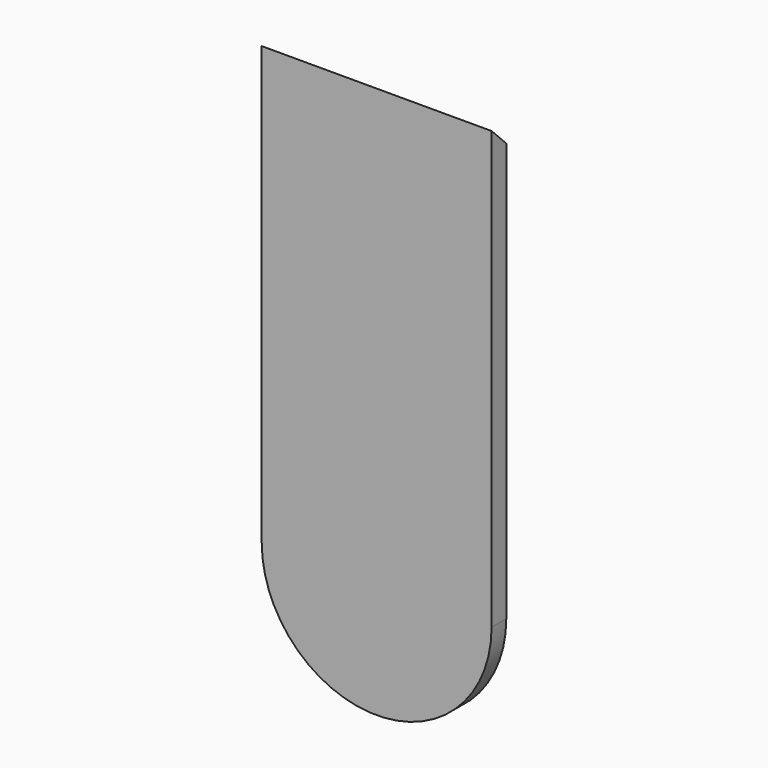
from build123d import *

# Parameters (mm, degrees)
F1_DEPTH = 20
F0_W     = 250
F0_H     = 475
F2_DEPTH = 20
F3_SIZE  = 19.99999


# Not quite as in the source:
# - a fillet or chamfer is up to 0.001 mm smaller than in the source, because OpenCascade refuses the exact size


with BuildPart() as f1:
    # F0 (on Front) → F1 (new body)
    with BuildSketch(Plane.XZ):
        with BuildLine():
            Line((123.788267374, 0), (-126.211732626, 0))
            ThreePointArc((-126.211732626, 0), (-1.211732626, -125), (123.788267374, 0))
        make_face()
    extrude(amount=F1_DEPTH)

    # F0 (on Front) → F2 (join)
    with BuildSketch(Plane.XZ):
        with Locations((-1.211732626, 237.5)):
            Rectangle(F0_W, F0_H)
    extrude(amount=F2_DEPTH)

    # F3 (size 20 in the source; OpenCascade refuses exactly that, so slightly less here)
    f3_edges = [f1.edges().sort_by_distance(p)[0] for p in [
        (-1.211733, 0, 475),
    ]]
    chamfer(f3_edges, length=F3_SIZE)


solid = f1.part
